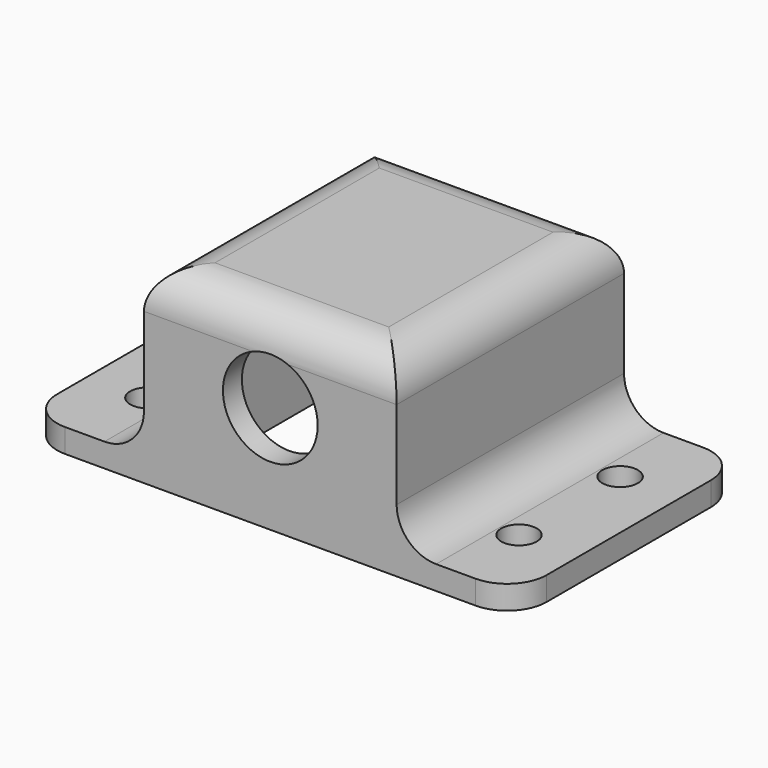
from build123d import *

# Parameters (mm, degrees)
F0_W        = 32
F0_H        = 21.1520095187
F0_R        = 6
F1_DEPTH    = 30
F2_T        = -2.5
F3_DEPTH    = 3
F4_W        = 32
F4_H        = 21.1520095187
F4_R        = 3
F5_DEPTH    = 3
F6_R        = 2.25
F7_DEPTH    = 3
F8_T1_DEPTH = 36
F8_T3_DEPTH = 61
F8_T5_DEPTH = 57
F8_T7_DEPTH = 28


# Not quite as in the source:
# - a fillet or chamfer that OpenCascade refuses, or shapes differently, is made with other operations: its cross-section is extruded or revolved along the edge and cut away or added
# - a feature names something its author has since deleted; it is built from what else it names


with BuildPart() as f1:
    # F0 (on Front) → F1 (new body)
    with BuildSketch(Plane.XZ):
        Rectangle(F0_W, F0_H)
        Circle(F0_R, mode=Mode.SUBTRACT)
        Circle(F0_R)
    extrude(amount=-F1_DEPTH)

    # F2
    f2_openings = [f1.faces().sort_by_distance(p)[0] for p in [
        (0, 0, 0),
        (0, 30, 0),
        (0, 15, -10.576005),
    ]]
    offset(amount=F2_T, openings=f2_openings)

    # F0 (on Front) → F3 (join)
    with BuildSketch(Plane.XZ):
        Rectangle(F0_W, F0_H)
        Circle(F0_R, mode=Mode.SUBTRACT)
    extrude(amount=F3_DEPTH)

    # F4 (on face) → F5 (join)
    with BuildSketch(Plane(origin=(0, 30, 0), x_dir=(-1, 0, 0), z_dir=(0, 1, 0))):
        Rectangle(F4_W, F4_H)
        Circle(F4_R, mode=Mode.SUBTRACT)
    extrude(amount=F5_DEPTH)

    # F6 (on face) → F7 (join)
    with BuildSketch(Plane(origin=(0, 0, -10.5760047594), x_dir=(1, 0, 0), z_dir=(0, 0, -1))):
        Polygon((-16, 3), (-16, 0), (-13.5, 0), (13.5, 0), (16, 0), (16, 3), align=None)
        Polygon((-16, -33), (-16, 0), (-16, 3), (-31, 3), (-31, -33), align=None)
        with Locations((-23.5, -23)):
            Circle(F6_R, mode=Mode.SUBTRACT)
        with Locations((-23.5, -7)):
            Circle(F6_R, mode=Mode.SUBTRACT)
        Polygon((-13.5, 0), (-16, 0), (-16, -33), (16, -33), (16, 0), (13.5, 0), (13.5, -30), (-13.5, -30), align=None)
        Polygon((31, 3), (16, 3), (16, 0), (16, -33), (31, -33), align=None)
        with Locations((23.5, -23)):
            Circle(F6_R, mode=Mode.SUBTRACT)
        with Locations((23.5, -7)):
            Circle(F6_R, mode=Mode.SUBTRACT)
    extrude(amount=F7_DEPTH)

    # F8: fillet of radius 5 on 10 edges, made by hand

    # F8_s2 → F8_t1 (join)
    with BuildSketch(Plane.XZ.offset(-33)):
        with BuildLine():
            ThreePointArc((-16, -5.5760047594), (-17.4644660941, -9.1115386653), (-21, -10.5760047594))
            Line((-21, -10.5760047594), (-16, -10.5760047594))
            Line((-16, -10.5760047594), (-16, -5.5760047594))
        make_face()
        with BuildLine():
            ThreePointArc((16, -5.5760047594), (17.4644660941, -9.1115386653), (21, -10.5760047594))
            Line((21, -10.5760047594), (16, -10.5760047594))
            Line((16, -10.5760047594), (16, -5.5760047594))
        make_face()
    extrude(amount=F8_T1_DEPTH)

    # F8_s4 → F8_t3 (cut)
    with BuildSketch(Plane.XZ.offset(-45.5)):
        with BuildLine():
            ThreePointArc((-11, 10.5760047594), (-14.5355339059, 9.1115386653), (-16, 5.5760047594))
            Line((-16, 5.5760047594), (-16, 10.5760047594))
            Line((-16, 10.5760047594), (-11, 10.5760047594))
        make_face()
        with BuildLine():
            ThreePointArc((16, 5.5760047594), (14.5355339059, 9.1115386653), (11, 10.5760047594))
            Line((11, 10.5760047594), (16, 10.5760047594))
            Line((16, 10.5760047594), (16, 5.5760047594))
        make_face()
    extrude(amount=F8_T3_DEPTH, mode=Mode.SUBTRACT)

    # F8_s6 → F8_t5 (cut)
    with BuildSketch(Plane.YZ.offset(-28.5)):
        with BuildLine():
            ThreePointArc((-3, 5.5760047594), (-1.5355339059, 9.1115386653), (2, 10.5760047594))
            Line((2, 10.5760047594), (-3, 10.5760047594))
            Line((-3, 10.5760047594), (-3, 5.5760047594))
        make_face()
        with BuildLine():
            ThreePointArc((28, 10.5760047594), (31.5355339059, 9.1115386653), (33, 5.5760047594))
            Line((33, 5.5760047594), (33, 10.5760047594))
            Line((33, 10.5760047594), (28, 10.5760047594))
        make_face()
    extrude(amount=F8_T5_DEPTH, mode=Mode.SUBTRACT)

    # F8_s8 → F8_t7 (cut)
    with BuildSketch(Plane.XY.offset(-26.0760047594)):
        with BuildLine():
            ThreePointArc((26, -3), (29.5355339059, -1.5355339059), (31, 2))
            Line((31, 2), (31, -3))
            Line((31, -3), (26, -3))
        make_face()
        with BuildLine():
            ThreePointArc((26, 33), (29.5355339059, 31.5355339059), (31, 28))
            Line((31, 28), (31, 33))
            Line((31, 33), (26, 33))
        make_face()
        with BuildLine():
            ThreePointArc((-26, -3), (-29.5355339059, -1.5355339059), (-31, 2))
            Line((-31, 2), (-31, -3))
            Line((-31, -3), (-26, -3))
        make_face()
        with BuildLine():
            ThreePointArc((-26, 33), (-29.5355339059, 31.5355339059), (-31, 28))
            Line((-31, 28), (-31, 33))
            Line((-31, 33), (-26, 33))
        make_face()
    extrude(amount=F8_T7_DEPTH, mode=Mode.SUBTRACT)


solid = f1.part
